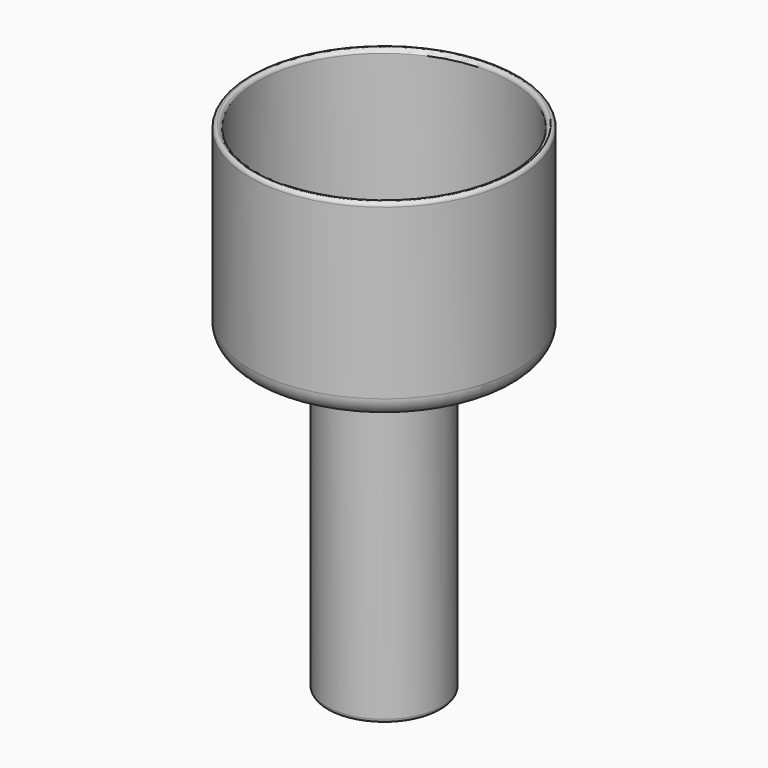
from build123d import *

# Parameters (mm, degrees)
F2_R = 0.99999
F3_R = 5
F4_R = 5


# Not quite as in the source:
# - a fillet or chamfer is up to 0.001 mm smaller than in the source, because OpenCascade refuses the exact size


with BuildPart() as f1:
    # F0 (on Front) → F1 (revolve)
    with BuildSketch(Plane.XZ):
        Polygon((-33, 57.2000007471), (-35, 57.2000007471), (-35, 7.2000007471), (-15, 7.2000007471), (-15, -72.7999992529), (-13, -72.7999992529), (-13, 9.2000007471), (-33, 9.2000007471), align=None)
    revolve(axis=Axis((0, 0, -7.7999992529), (0, 0, 1)))

    # F2 (radius 1 in the source; OpenCascade refuses exactly that, so slightly less here)
    f2_edges = [f1.edges().sort_by_distance(p)[0] for p in [
        (35, 0, 57.200001),
        (33, 0, 57.200001),
        (15, 0, -72.799999),
        (13, 0, -72.799999),
    ]]
    fillet(f2_edges, radius=F2_R)

    # F3
    f3_edges = [f1.edges().sort_by_distance(p)[0] for p in [
        (15, 0, 7.200001),
        (35, 0, 7.200001),
    ]]
    fillet(f3_edges, radius=F3_R)

    # F4
    f4_edges = [f1.edges().sort_by_distance(p)[0] for p in [
        (13, 0, 9.200001),
        (33, 0, 9.200001),
    ]]
    fillet(f4_edges, radius=F4_R)


solid = f1.part
